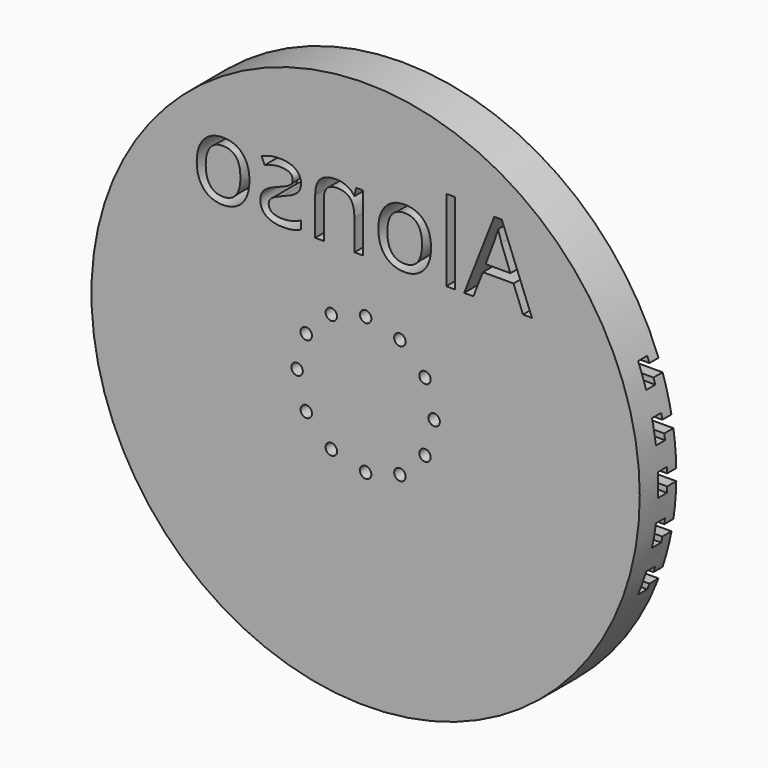
from build123d import *

# Parameters (mm, degrees)
F0_R         = 152.4
F1_DEPTH     = 25.4
F3_D         = 6.35
F3_DEPTH     = 9.525
F3_TIP       = 1.9077324654
F7_DEPTH     = 304.8
F8_TEXT_SIZE = 59.5663777656
F9_DEPTH     = 25.4


# Not quite as in the source:
# - Text() gives the source's letters only with a copy of the font that has no kerning and outlines rounded to 1/6400 em; it was checked with that copy


with BuildPart() as f1:
    # F0 (on Front) → F1 (new body)
    with BuildSketch(Plane.XZ):
        Circle(F0_R)
    extrude(amount=F1_DEPTH)

    # F3
    with Locations(Plane.XZ.offset(25.4)):
        with Locations((-19.05, 32.9955678842), (0, 38.1), (19.05, 32.9955678842), (32.9955678842, 19.05), (38.1, 0), (32.9955678842, -19.05), (19.05, -32.9955678842), (0, -38.1), (-19.05, -32.9955678842), (-32.9955678842, -19.05), (-32.9955678842, 19.05), (-38.1, 0)):
            Hole(F3_D / 2, depth=F3_DEPTH)
            with Locations((0, 0, -(F3_DEPTH + F3_TIP / 2))):  # 118° drill point
                Cone(0, F3_D / 2, F3_TIP, mode=Mode.SUBTRACT)

    # F6 (on offset) → F7 (cut)
    with BuildSketch(Plane.YZ.offset(152.4)):
        Polygon((-6.35, -3.175), (0, -3.175), (0, 3.175), (-6.35, 3.175), (-6.35, 6.35), (-12.7, 6.35), (-12.7, -6.35), (-6.35, -6.35), align=None)
        Polygon((-6.35, -53.975), (0, -53.975), (0, -47.625), (-6.35, -47.625), (-6.35, -44.45), (-12.7, -44.45), (-12.7, -57.15), (-6.35, -57.15), align=None)
        Polygon((-6.35, -28.575), (0, -28.575), (0, -22.225), (-6.35, -22.225), (-6.35, -19.05), (-12.7, -19.05), (-12.7, -31.75), (-6.35, -31.75), align=None)
        Polygon((-6.35, 22.225), (0, 22.225), (0, 28.575), (-6.35, 28.575), (-6.35, 31.75), (-12.7, 31.75), (-12.7, 28.575), (-12.7, 19.05), (-6.35, 19.05), align=None)
        Polygon((-6.35, 47.625), (0, 47.625), (0, 53.975), (-6.35, 53.975), (-6.35, 57.15), (-12.7, 57.15), (-12.7, 44.45), (-6.35, 44.45), align=None)
    extrude(amount=-F7_DEPTH, mode=Mode.SUBTRACT)

    # F8 (on face) → F9 (cut)
    with BuildSketch(Plane(origin=(0, 0, 0), x_dir=(-1, 0, 0), z_dir=(0, 1, 0))):
        with Locations((-92.4694687128, 67.5485357642)):
            Text('Alonso', F8_TEXT_SIZE, font='Open Sans', text_align=(TextAlign.LEFT, TextAlign.BOTTOM))
    extrude(amount=-F9_DEPTH, mode=Mode.SUBTRACT)


solid = f1.part
